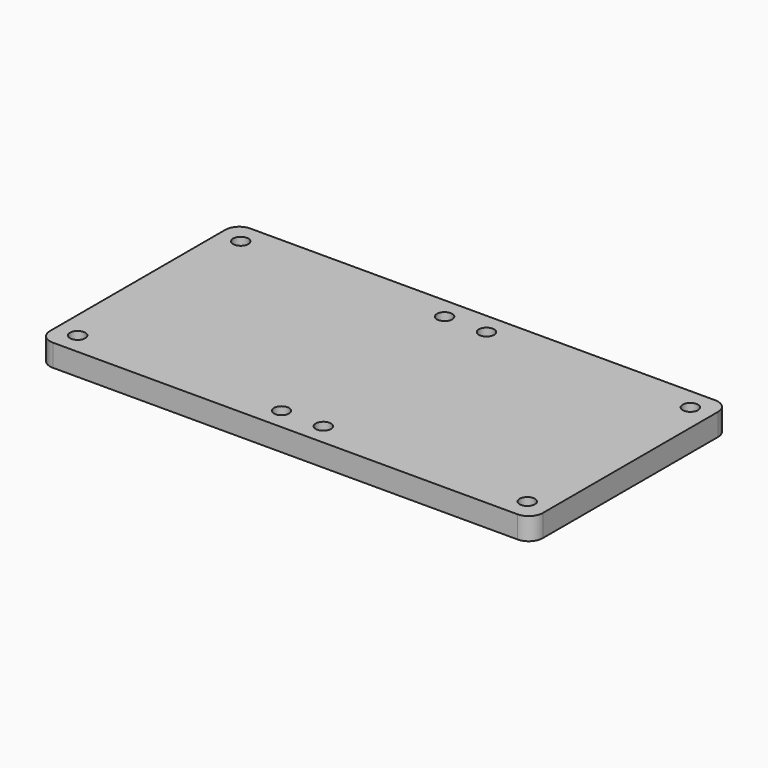
from build123d import *

# Parameters (mm, degrees)
F1_W     = 70.58
F1_H     = 35.38
F2_DEPTH = 3.175
F0_R     = 1.09
F3_DEPTH = 3.176
F4_R     = 2


# Not quite as in the source:
# - a length typed as a fraction of an inch, garbled in the dataset ("3 / 203.2 mm" for 3/8 in), is restored


with BuildPart() as f2:
    # F1 (on Top) → F2 (new body)
    with BuildSketch(Plane.XY):
        Rectangle(F1_W, F1_H)
    extrude(amount=F2_DEPTH)

    # F0 (on Top) → F3 (cut, through all)
    with BuildSketch(Plane.XY):
        with Locations((-3, 14.6)):
            Circle(F0_R)
        with Locations((-3, -14.6)):
            Circle(F0_R)
        with Locations((-32.2, -14.6)):
            Circle(F0_R)
        with Locations((32.2, 14.6)):
            Circle(F0_R)
        with Locations((32.2, -14.6)):
            Circle(F0_R)
        with Locations((3, -14.6)):
            Circle(F0_R)
        with Locations((-32.2, 14.6)):
            Circle(F0_R)
        with Locations((3, 14.6)):
            Circle(F0_R)
    extrude(amount=F3_DEPTH, mode=Mode.SUBTRACT)

    # F4
    f4_edges = [f2.edges().sort_by_distance(p)[0] for p in [
        (-35.29, -17.69, 1.5875),
        (-35.29, 17.69, 1.5875),
        (35.29, 17.69, 1.5875),
        (35.29, -17.69, 1.5875),
    ]]
    fillet(f4_edges, radius=F4_R)


solid = f2.part
